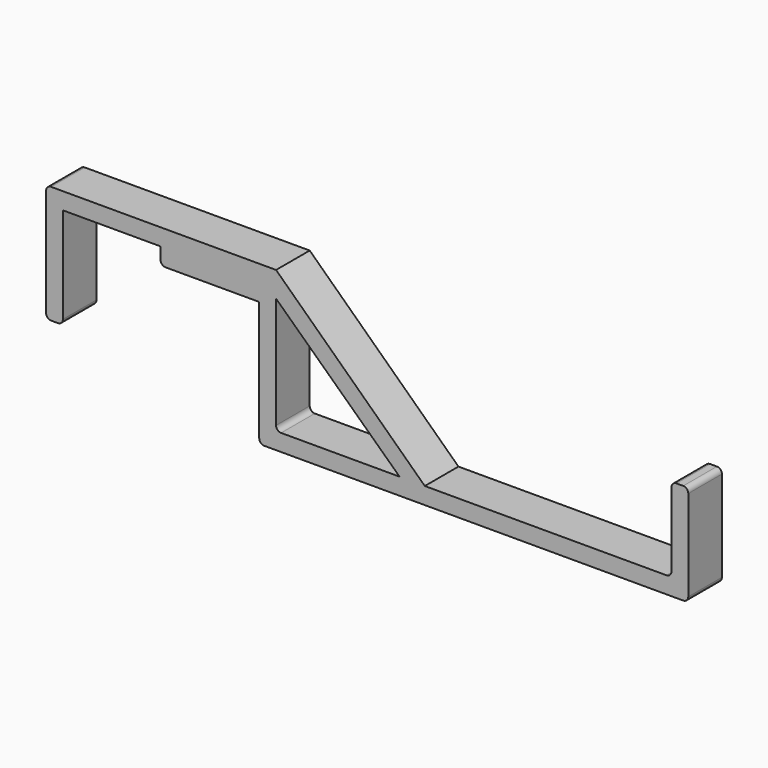
from build123d import *

# Parameters (mm, degrees)
F0_W     = 14.9098
F0_H     = 2.54
F0_W_2   = 2.54
F0_H_2   = 12.7
F1_DEPTH = 6.35
F2_R     = 0.762


with BuildPart() as f1:
    # F0 (on Front) → F1 (new body)
    with BuildSketch(Plane.XZ):
        Polygon((0, -2.54), (0, 0), (-2.54, 0), (-2.54, -17.78), (0, -17.78), align=None)
        Polygon((29.6418, 0), (0, 0), (0, -2.54), (14.732, -2.54), (29.6418, -2.54), align=None)
        with Locations((22.1869, -3.81)):
            Rectangle(F0_W, F0_H)
        Polygon((32.1818, 0), (29.6418, 0), (29.6418, -2.54), (29.6418, -5.08), (29.6418, -23.9522), (32.1818, -23.9522), (32.1818, -21.4122), (32.1818, -3.81), align=None)
        Polygon((91.8718, -21.4122), (54.6354, -21.4122), (50.8254, -21.4122), (32.1818, -21.4122), (32.1818, -23.9522), (94.4118, -23.9522), (94.4118, -21.4122), align=None)
        with Locations((93.1418, -15.0622)):
            Rectangle(F0_W_2, F0_H_2)
        Polygon((54.6354, -21.4122), (32.1818, 0), (32.1818, -3.81), (50.8254, -21.4122), align=None)
    extrude(amount=F1_DEPTH)

    # F2
    f2_edges = [f1.edges().sort_by_distance(p)[0] for p in [
        (-2.54, -3.175, -17.78),
        (0, -3.175, -17.78),
        (-2.54, -3.175, 0),
        (32.1818, -3.175, -21.4122),
        (14.732, -3.175, -5.08),
        (29.6418, -3.175, -23.9522),
        (94.4118, -3.175, -23.9522),
        (94.4118, -3.175, -8.7122),
        (91.8718, -3.175, -8.7122),
        (91.8718, -3.175, -21.4122),
    ]]
    fillet(f2_edges, radius=F2_R)


solid = f1.part
